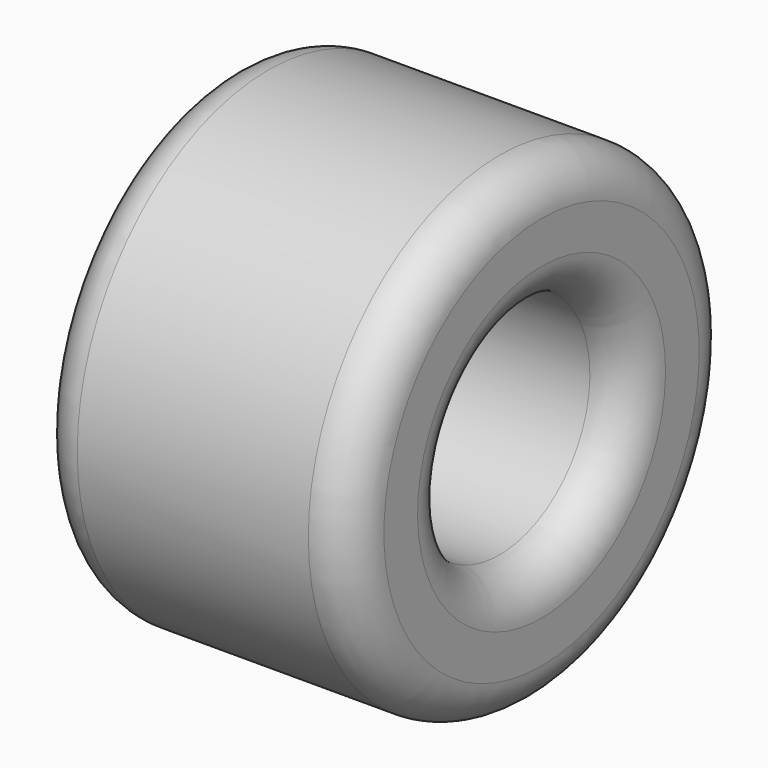
from build123d import *


# Not quite as in the source:
# - the program builds the solid bodies; features that only make, move or delete a surface that nothing else refers to are left out


with BuildPart() as f3:
    # F0 (on Front) → F3 (revolve)
    with BuildSketch(Plane.XZ):
        with BuildLine():
            Line((125.4684708416, -176.5307388092), (-153.9315291584, -176.5307388092))
            ThreePointArc((-153.9315291584, -176.5307388092), (-189.8525536426, -191.409714325), (-204.7315291584, -227.3307388092))
            Line((-204.7315291584, -227.3307388092), (-204.7315291584, -278.1307388092))
            ThreePointArc((-204.7315291584, -278.1307388092), (-189.8525536426, -314.0517632935), (-153.9315291584, -328.9307388092))
            Line((-153.9315291584, -328.9307388092), (125.4684708416, -328.9307388092))
            ThreePointArc((125.4684708416, -328.9307388092), (161.3894953259, -314.0517632935), (176.2684708416, -278.1307388092))
            Line((176.2684708416, -278.1307388092), (176.2684708416, -227.3307388092))
            ThreePointArc((176.2684708416, -227.3307388092), (161.3894953259, -191.409714325), (125.4684708416, -176.5307388092))
        make_face()
    revolve(axis=Axis((3.1946003437, 0, -465.563416481), (1, 0, 0)))


solid = f3.part
